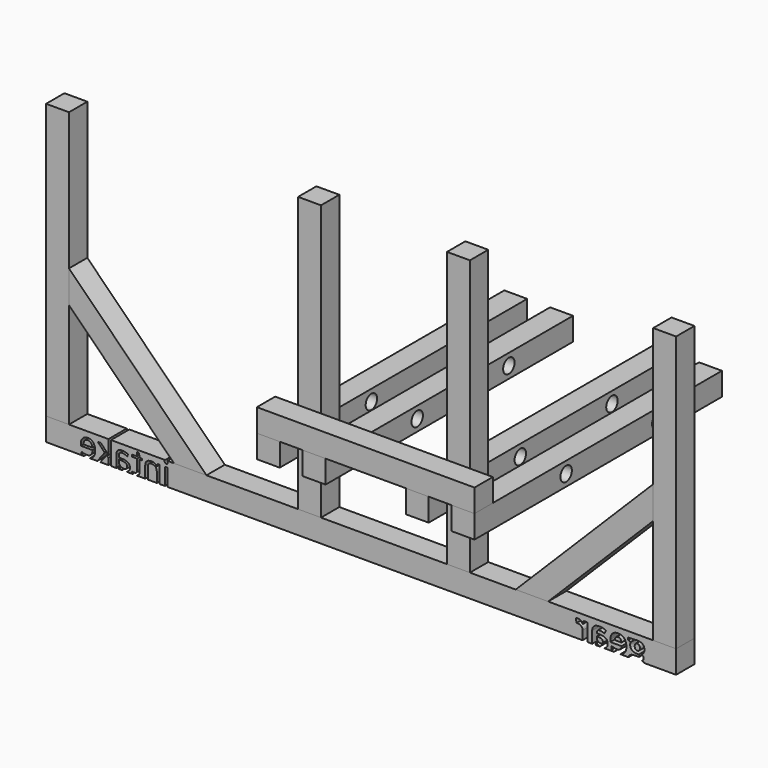
from build123d import *

# Parameters (mm, degrees)
F3_W           = 25.4
F3_H           = 25.4
F4_DEPTH       = 304.8
F5_W           = 698.5
F5_H           = 25.4
F6_DEPTH       = 12.7
F7_TEXT_SIZE   = 35.2777777778
F8_DEPTH       = 25.401
F10_DEPTH      = 12.7
F11_W          = 25.4
F11_H          = 25.4
F12_DEPTH      = 38.1
F12_DEPTH_BACK = 304.8
F13_W          = 241.3
F13_H          = 25.4
F14_DEPTH      = 25.4
F15_R          = 7.9375
F16_DEPTH      = 495.3010001
F17_R          = 7.9375
F18_DEPTH      = 495.3010001


# Not quite as in the source:
# - Text() gives the source's letters only with a copy of the font that has no kerning and outlines rounded to 1/6400 em; it was checked with that copy


with BuildPart() as f4:
    # F3 (on Top) → F4 (new body)
    with BuildSketch(Plane.XY):
        with Locations((-336.55, 0)):
            Rectangle(F3_W, F3_H)
    extrude(amount=F4_DEPTH)


with BuildPart() as f4b:
    # F3 (on Top) → F4, piece 2 (new body)
    with BuildSketch(Plane.XY):
        with Locations((-57.15, 0)):
            Rectangle(F3_W, F3_H)
    extrude(amount=F4_DEPTH)


with BuildPart() as f4c:
    # F3 (on Top) → F4, piece 3 (new body)
    with BuildSketch(Plane.XY):
        with Locations((107.95, 0)):
            Rectangle(F3_W, F3_H)
    extrude(amount=F4_DEPTH)


with BuildPart() as f4d:
    # F3 (on Top) → F4, piece 4 (new body)
    with BuildSketch(Plane.XY):
        with Locations((336.55, 0)):
            Rectangle(F3_W, F3_H)
    extrude(amount=F4_DEPTH)


with BuildPart() as f6:
    # F5 (on Front) → F6 (new body, symmetric)
    with BuildSketch(Plane.XZ):
        with Locations((0, -12.7)):
            Rectangle(F5_W, F5_H)
    extrude(amount=F6_DEPTH, both=True)

    # F7 (on face) → F8 (cut, through all)
    with BuildSketch(Plane(origin=(0, 12.7, 0), x_dir=(-1, 0, 0), z_dir=(0, 1, 0))):
        with Locations((-315.6553208828, -25.4)):
            Text('gear', F7_TEXT_SIZE, font='Open Sans', font_style=FontStyle.BOLD, text_align=(TextAlign.LEFT, TextAlign.BOTTOM))
        with Locations((211.6142958403, -25.4)):
            Text('intake', F7_TEXT_SIZE, font='Open Sans', text_align=(TextAlign.LEFT, TextAlign.BOTTOM))
    extrude(amount=-F8_DEPTH, mode=Mode.SUBTRACT)


with BuildPart() as f10:
    # F9 (on Front) → F10 (new body, symmetric)
    with BuildSketch(Plane.XZ):
        Polygon((323.85, 152.4), (171.45, 0), (207.3710244843, 0), (323.85, 116.4789755157), align=None)
    extrude(amount=F10_DEPTH, both=True)


with BuildPart() as f10b:
    # F9 (on Front) → F10, piece 2 (new body, symmetric)
    with BuildSketch(Plane.XZ):
        Polygon((-207.3710244843, 0), (-171.45, 0), (-323.85, 152.4), (-323.85, 116.4789755157), align=None)
    extrude(amount=F10_DEPTH, both=True)


with BuildPart() as f12:
    # F11 (on Front) → F12 (new body, two sides)
    with BuildSketch(Plane.XZ) as f12_sk:
        with Locations((133.35, 63.5)):
            Rectangle(F11_W, F11_H)
    extrude(amount=F12_DEPTH)
    extrude(f12_sk.sketch, amount=-F12_DEPTH_BACK)


with BuildPart() as f12b:
    # F11 (on Front) → F12, piece 2 (new body, two sides)
    with BuildSketch(Plane.XZ) as f12_2_sk:
        with Locations((82.55, 63.5)):
            Rectangle(F11_W, F11_H)
    extrude(amount=F12_DEPTH)
    extrude(f12_2_sk.sketch, amount=-F12_DEPTH_BACK)


with BuildPart() as f12c:
    # F11 (on Front) → F12, piece 3 (new body, two sides)
    with BuildSketch(Plane.XZ) as f12_3_sk:
        with Locations((-31.75, 63.5)):
            Rectangle(F11_W, F11_H)
    extrude(amount=F12_DEPTH)
    extrude(f12_3_sk.sketch, amount=-F12_DEPTH_BACK)


with BuildPart() as f12d:
    # F11 (on Front) → F12, piece 4 (new body, two sides)
    with BuildSketch(Plane.XZ) as f12_4_sk:
        with Locations((-82.55, 63.5)):
            Rectangle(F11_W, F11_H)
    extrude(amount=F12_DEPTH)
    extrude(f12_4_sk.sketch, amount=-F12_DEPTH_BACK)


with BuildPart() as f14:
    # F13 (on face) → F14 (new body)
    with BuildSketch(Plane.XY.offset(76.2)):
        with Locations((25.4, -25.4)):
            Rectangle(F13_W, F13_H)
    extrude(amount=F14_DEPTH)


with BuildPart() as f16_tool:
    # F15 (on face) → F16 (new body, through all)
    with BuildSketch(Plane.YZ.offset(146.05)):
        with Locations((215.9, 63.5)):
            Circle(F15_R)
    extrude(amount=-F16_DEPTH)


with BuildPart() as f12_1:
    add(f12.part)

    # F16: cut by f16_tool
    add(f16_tool.part, mode=Mode.SUBTRACT)


with BuildPart() as f12b_1:
    add(f12b.part)

    # F16: cut by f16_tool
    add(f16_tool.part, mode=Mode.SUBTRACT)


with BuildPart() as f12c_1:
    add(f12c.part)

    # F16: cut by f16_tool
    add(f16_tool.part, mode=Mode.SUBTRACT)


with BuildPart() as f12d_1:
    add(f12d.part)

    # F16: cut by f16_tool
    add(f16_tool.part, mode=Mode.SUBTRACT)


with BuildPart() as f18_tool:
    # F17 (on face) → F18 (new body, through all)
    with BuildSketch(Plane.YZ.offset(146.05)):
        with Locations((88.9, 63.5)):
            Circle(F17_R)
    extrude(amount=-F18_DEPTH)


with BuildPart() as f12_2:
    add(f12_1.part)

    # F18: cut by f18_tool
    add(f18_tool.part, mode=Mode.SUBTRACT)


with BuildPart() as f12b_2:
    add(f12b_1.part)

    # F18: cut by f18_tool
    add(f18_tool.part, mode=Mode.SUBTRACT)


with BuildPart() as f12c_2:
    add(f12c_1.part)

    # F18: cut by f18_tool
    add(f18_tool.part, mode=Mode.SUBTRACT)


with BuildPart() as f12d_2:
    add(f12d_1.part)

    # F18: cut by f18_tool
    add(f18_tool.part, mode=Mode.SUBTRACT)


solid = Compound([f4.part, f4b.part, f4c.part, f4d.part, f6.part, f10.part, f10b.part, f14.part, f12_2.part, f12b_2.part, f12c_2.part, f12d_2.part])
